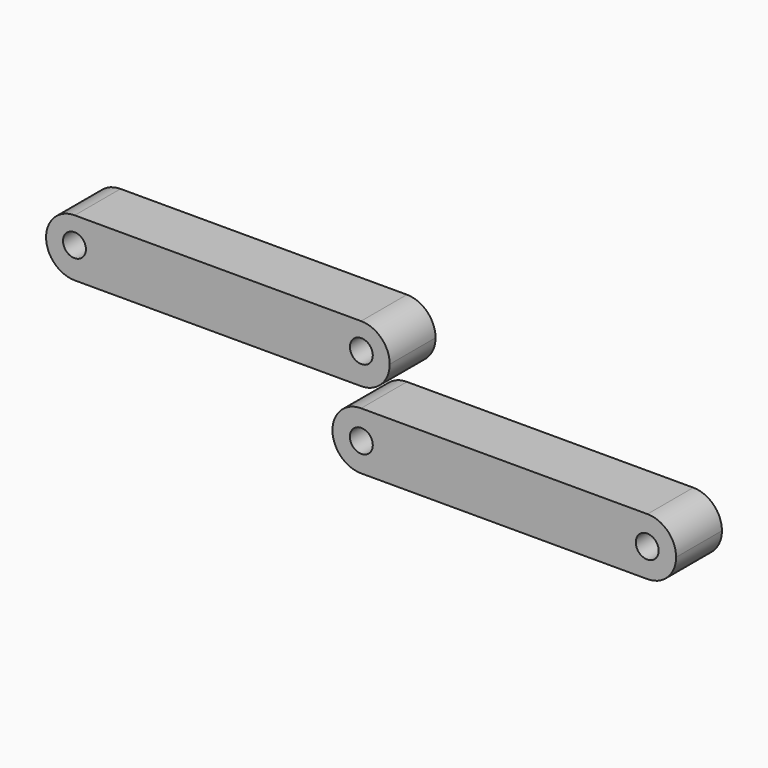
from build123d import *

# Parameters (mm, degrees)
F0_W     = 60
F0_H     = 10
F0_R     = 2
F1_DEPTH = 10
F2_R     = 4.99999
F2_2_R   = 4.99999


# Not quite as in the source:
# - a fillet or chamfer is up to 0.001 mm smaller than in the source, because OpenCascade refuses the exact size


with BuildPart() as f1:
    # F0 (on Front) → F1 (new body)
    with BuildSketch(Plane.XZ):
        with Locations((-787.4018650077, -227.7252674103)):
            Rectangle(F0_W, F0_H)
        with Locations((-812.4446220431, -227.3237803578)):
            Circle(F0_R, mode=Mode.SUBTRACT)
        with Locations((-762.3591079723, -227.3237803578)):
            Circle(F0_R, mode=Mode.SUBTRACT)
    extrude(amount=F1_DEPTH)

    # F2 (radius 5 in the source; OpenCascade refuses exactly that, so slightly less here)
    f2_edges = [f1.edges().sort_by_distance(p)[0] for p in [
        (-757.401865, -5, -222.725267),
        (-757.401865, -5, -232.725267),
        (-817.401865, -5, -222.725267),
        (-817.401865, -5, -232.725267),
    ]]
    fillet(f2_edges, radius=F2_R)


with BuildPart() as f1b:
    # F0 (on Front) → F1, piece 2 (new body)
    with BuildSketch(Plane.XZ):
        with Locations((-737.4018650077, -241.1261898279)):
            Rectangle(F0_W, F0_H)
        with Locations((-762.3591079723, -241.1261898279)):
            Circle(F0_R, mode=Mode.SUBTRACT)
        with Locations((-712.4446220431, -241.1261898279)):
            Circle(F0_R, mode=Mode.SUBTRACT)
    extrude(amount=F1_DEPTH)

    # F2#2 (radius 5 in the source; OpenCascade refuses exactly that, so slightly less here)
    f2_2_edges = [f1b.edges().sort_by_distance(p)[0] for p in [
        (-767.401865, -5, -236.12619),
        (-767.401865, -5, -246.12619),
        (-707.401865, -5, -236.12619),
        (-707.401865, -5, -246.12619),
    ]]
    fillet(f2_2_edges, radius=F2_2_R)


solid = Compound([f1.part, f1b.part])
